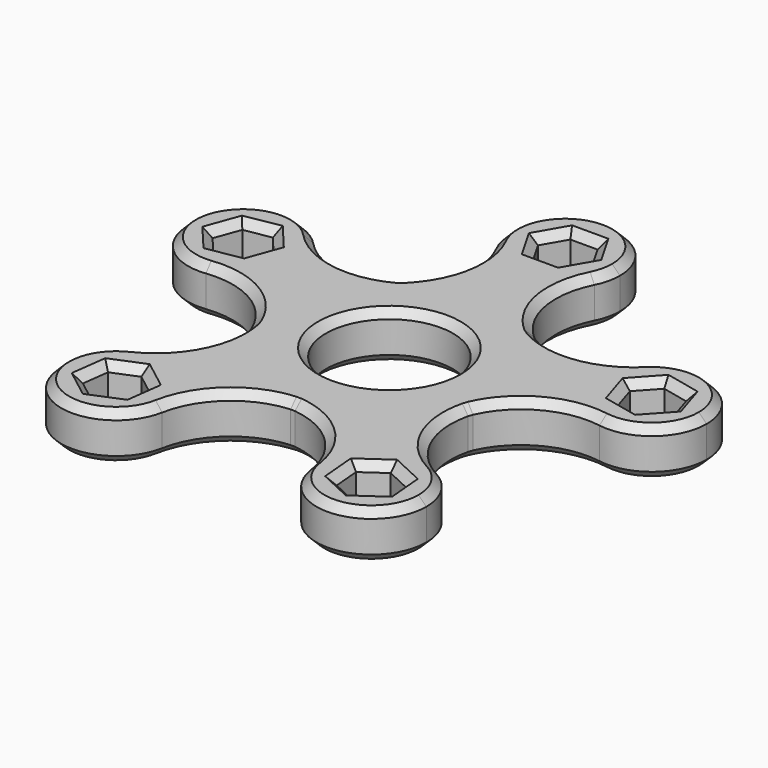
from build123d import *

# Parameters (mm, degrees)
F0_R        = 8.1
F1_DEPTH    = 6
F3_DEPTH    = 25
F4_C1_SIZE  = 1
F4_C2_SIZE  = 1
F4_C3_SIZE  = 1
F4_C4_SIZE  = 1
F4_C5_SIZE  = 1
F4_C6_SIZE  = 1
F4_C7_SIZE  = 1
F4_C8_SIZE  = 1
F4_C9_SIZE  = 1
F4_C10_SIZE = 1
F4_C11_SIZE = 1
F4_C12_SIZE = 1
F4_C13_SIZE = 1
F4_C14_SIZE = 1
F4_C15_SIZE = 1
F4_C16_SIZE = 1
F4_C17_SIZE = 1
F4_C18_SIZE = 1
F4_C19_SIZE = 1
F4_C20_SIZE = 1
F4_C21_SIZE = 1
F4_C22_SIZE = 1
F4_C23_SIZE = 1
F4_C24_SIZE = 1
F4_C25_SIZE = 1
F4_C26_SIZE = 1
F4_C27_SIZE = 1
F4_C28_SIZE = 1
F4_C29_SIZE = 1
F4_C30_SIZE = 1
F4_C31_SIZE = 1
F4_C32_SIZE = 1
F4_C33_SIZE = 1
F4_C34_SIZE = 1
F4_C35_SIZE = 1
F4_C36_SIZE = 1
F4_C37_SIZE = 1
F4_C38_SIZE = 1
F4_C39_SIZE = 1
F4_C40_SIZE = 1
F4_C41_SIZE = 1
F4_C42_SIZE = 1
F4_C43_SIZE = 1
F4_C44_SIZE = 1
F4_C45_SIZE = 1
F4_C46_SIZE = 1
F4_C47_SIZE = 1
F4_C48_SIZE = 1
F4_C49_SIZE = 1
F4_C50_SIZE = 1
F4_C51_SIZE = 1
F4_C52_SIZE = 1
F4_C53_SIZE = 1
F4_C54_SIZE = 1
F4_C55_SIZE = 1
F4_C56_SIZE = 1
F4_C57_SIZE = 1
F4_C58_SIZE = 1
F4_C59_SIZE = 1
F4_C60_SIZE = 1
F4_C61_SIZE = 1
F4_C62_SIZE = 0.9999
F4_C63_SIZE = 1
F4_C64_SIZE = 1
F4_C65_SIZE = 0.9999
F4_C66_SIZE = 0.9999
F4_C67_SIZE = 0.9999
F4_C68_SIZE = 0.9999
F4_C69_SIZE = 1
F4_C70_SIZE = 1
F4_C71_SIZE = 1
F4_C72_SIZE = 1
F4_C73_SIZE = 1
F4_C74_SIZE = 1
F4_C75_SIZE = 0.9999
F4_C76_SIZE = 0.9999
F4_C77_SIZE = 0.9999
F4_C78_SIZE = 0.9999
F4_C79_SIZE = 0.9999
F4_C80_SIZE = 0.9999


# Not quite as in the source:
# - a fillet or chamfer is up to 0.001 mm smaller than in the source, because OpenCascade refuses the exact size


with BuildPart() as f1:
    # F0 (on Top) → F1 (new body)
    with BuildSketch(Plane.XY):
        with BuildLine():
            ThreePointArc((14.2942212748, -4.5470032051), (14.8225051716, -2.3007260678), (15, 0))
            ThreePointArc((15, 0), (13.444632763, 6.6514547182), (9.1010866843, 11.9235154701))
            ThreePointArc((9.1010866843, 11.9235154701), (8.8696447255, 12.096669064), (8.6349092686, 12.2653308934))
            ThreePointArc((8.6349092686, 12.2653308934), (0.0381987951, 14.9999513617), (-8.5723280263, 12.3091507509))
            ThreePointArc((-8.5723280263, 12.3091507509), (-8.6036465453, 12.2872806643), (-8.6349092686, 12.2653308934))
            ThreePointArc((-8.6349092686, 12.2653308934), (-14.1084083641, 5.0943903887), (-14.4789538376, -3.9191702908))
            ThreePointArc((-14.4789538376, -3.9191702908), (-14.4007478158, -4.1974352105), (-14.3171944732, -4.4741415283))
            ThreePointArc((-14.3171944732, -4.4741415283), (-9.1314214351, -11.9003001044), (-0.6161262506, -14.9873409397))
            ThreePointArc((-0.6161262506, -14.9873409397), (-0.3272232755, -14.9964304062), (-0.0381987951, -14.9999513617))
            ThreePointArc((-0.0381987951, -14.9999513617), (8.6036465453, -12.2872806643), (14.1084083641, -5.0943903887))
            ThreePointArc((14.1084083641, -5.0943903887), (14.2039519424, -4.8215919795), (14.2942212748, -4.5470032051))
        make_face()
        Circle(F0_R, mode=Mode.SUBTRACT)
        with BuildLine():
            ThreePointArc((9.1010866843, 11.9235154701), (13.444632763, 6.6514547182), (15, 0))
            ThreePointArc((15, 0), (14.8225051716, -2.3007260678), (14.2942212748, -4.5470032051))
            ThreePointArc((14.2942212748, -4.5470032051), (18.9028221791, 0.3997534781), (25.5715973454, 1.5119772693))
            ThreePointArc((25.5715973454, 1.5119772693), (20.0280559657, 6.3148217896), (21.8142607752, 13.4287264061))
            ThreePointArc((21.8142607752, 13.4287264061), (15.7135746063, 10.5147545037), (9.1010866843, 11.9235154701))
        make_face()
        with BuildLine():
            ThreePointArc((-8.5723280263, 12.3091507509), (0.0381987951, 14.9999513617), (8.6349092686, 12.2653308934))
            ThreePointArc((8.6349092686, 12.2653308934), (5.302936588, 18.1481501185), (6.2475292735, 24.8427261796))
            ThreePointArc((6.2475292735, 24.8427261796), (0, 21), (-6.2475292735, 24.8427261796))
            ThreePointArc((-6.2475292735, 24.8427261796), (-5.2993669116, 18.1670506516), (-8.6062308953, 12.2909714987))
            ThreePointArc((-8.6062308953, 12.2909714987), (-8.589271136, 12.3000455997), (-8.5723280263, 12.3091507509))
        make_face()
        with BuildLine():
            ThreePointArc((33.704074621, 8.4197623861), (29.4217301436, 14.870680806), (21.8142607752, 13.4287264061))
            ThreePointArc((21.8142607752, 13.4287264061), (20.0280559657, 6.3148217896), (25.5715973454, 1.5119772693))
            ThreePointArc((25.5715973454, 1.5119772693), (31.2357773402, 3.0846269179), (33.704074621, 8.4197623861))
        make_face()
        with BuildLine():
            ThreePointArc((19.3668787275, -16.766534359), (14.7532626182, -11.8244547992), (14.1084083641, -5.0943903887))
            ThreePointArc((14.1084083641, -5.0943903887), (8.6036465453, -12.2872806643), (-0.0381987951, -14.9999513617))
            ThreePointArc((-0.0381987951, -14.9999513617), (6.0654399245, -17.90773374), (9.1315259752, -23.9334055124))
            ThreePointArc((9.1315259752, -23.9334055124), (12.0451051634, -17.2021929301), (19.3668787275, -16.766534359))
        make_face()
        with BuildLine():
            ThreePointArc((-8.6349092686, 12.2653308934), (-8.6036465453, 12.2872806643), (-8.5723280263, 12.3091507509))
            ThreePointArc((-8.5723280263, 12.3091507509), (-8.589271136, 12.3000455997), (-8.6062308953, 12.2909714987))
            ThreePointArc((-8.6062308953, 12.2909714987), (-8.6205583403, 12.2781380633), (-8.6349092686, 12.2653308934))
        make_face()
        with BuildLine():
            ThreePointArc((-6.2475292735, 24.8427261796), (0, 21), (6.2475292735, 24.8427261796))
            ThreePointArc((6.2475292735, 24.8427261796), (6.8092842838, 26.37714833), (7, 28))
            ThreePointArc((7, 28), (-1.62285167, 34.8092842838), (-6.2475292735, 24.8427261796))
        make_face()
        with BuildLine():
            ThreePointArc((23.0601402178, -22.9362572401), (22.0662691528, -19.3409248193), (19.3668787275, -16.766534359))
            ThreePointArc((19.3668787275, -16.766534359), (12.0451051634, -17.2021929301), (9.1315259752, -23.9334055124))
            ThreePointArc((9.1315259752, -23.9334055124), (16.5599903462, -29.9183879929), (23.0601402178, -22.9362572401))
        make_face()
        with BuildLine():
            ThreePointArc((-14.4789538376, -3.9191702908), (-14.1084083641, 5.0943903887), (-8.6349092686, 12.2653308934))
            ThreePointArc((-8.6349092686, 12.2653308934), (-8.6205583403, 12.2781380633), (-8.6062308953, 12.2909714987))
            ThreePointArc((-8.6062308953, 12.2909714987), (-15.2589532082, 11.1932732493), (-21.2077456136, 14.367469925))
            ThreePointArc((-21.2077456136, 14.367469925), (-19.8027247632, 12.1528467636), (-19.311393382, 9.5765640131))
            ThreePointArc((-19.311393382, 9.5765640131), (-21.0763861054, 4.9295543495), (-25.4813073287, 2.6259556121))
            ThreePointArc((-25.4813073287, 2.6259556121), (-18.8673938791, 1.2239025243), (-14.4789538376, -3.9191702908))
        make_face()
        with BuildLine():
            ThreePointArc((-10.1667952719, -23.5123146448), (-6.8407913445, -17.6261187719), (-0.6161262506, -14.9873409397))
            ThreePointArc((-0.6161262506, -14.9873409397), (-9.1314214351, -11.9003001044), (-14.3171944732, -4.4741415283))
            ThreePointArc((-14.3171944732, -4.4741415283), (-15.2549962555, -11.1696722613), (-20.0797917072, -15.9058049482))
            ThreePointArc((-20.0797917072, -15.9058049482), (-13.3198201709, -16.2876256526), (-10.0453200122, -22.2138935282))
            ThreePointArc((-10.0453200122, -22.2138935282), (-10.0757549906, -22.8659390854), (-10.1667952719, -23.5123146448))
        make_face()
        with BuildLine():
            ThreePointArc((-19.311393382, 9.5765640131), (-19.8027247632, 12.1528467636), (-21.2077456136, 14.367469925))
            ThreePointArc((-21.2077456136, 14.367469925), (-32.8892417275, 11.9707050164), (-25.4813073287, 2.6259556121))
            ThreePointArc((-25.4813073287, 2.6259556121), (-21.0763861054, 4.9295543495), (-19.311393382, 9.5765640131))
        make_face()
        with BuildLine():
            ThreePointArc((-20.0797917072, -15.9058049482), (-21.3066500153, -27.7673669102), (-10.1667952719, -23.5123146448))
            ThreePointArc((-10.1667952719, -23.5123146448), (-10.0757549906, -22.8659390854), (-10.0453200122, -22.2138935282))
            ThreePointArc((-10.0453200122, -22.2138935282), (-13.3198201709, -16.2876256526), (-20.0797917072, -15.9058049482))
        make_face()
    extrude(amount=F1_DEPTH)

    # F2 (on face) → F3 (cut)
    with BuildSketch(Plane.XY.offset(6)):
        Polygon((1.7320508076, 31), (-1.7320508076, 31), (-3.4641016151, 28), (-1.7320508076, 25), (1.7320508076, 25), (3.4641016151, 28), align=None)
        Polygon((30.0860631961, 7.6699935699), (29.0443877503, 10.9737659994), (25.6623991752, 11.7235348156), (23.3220860458, 9.1695312023), (24.3637614916, 5.8657587729), (27.7457500667, 5.1159899566), align=None)
        Polygon((16.362056567, -26.3871769027), (19.1996824867, -24.4002498432), (18.8977661375, -20.9493301805), (15.7582238686, -19.4853375774), (12.9205979489, -21.472264637), (13.2225142982, -24.9231842997), align=None)
        Polygon((-13.8449074315, -20.888239232), (-16.593164019, -18.7794277825), (-19.7935765997, -20.1050820787), (-20.245732593, -23.5395478243), (-17.4974760055, -25.6483592738), (-14.2970634248, -24.3227049776), align=None)
        Polygon((-24.0847117851, 6.9229082204), (-22.8999192542, 10.1780989458), (-25.1266008511, 12.8317547385), (-28.5380749789, 12.2302198058), (-29.7228675098, 8.9750290804), (-27.4961859129, 6.3213732877), align=None)
    extrude(amount=-F3_DEPTH, mode=Mode.SUBTRACT)

    # F4: chamfer of 1 on 100 edges, made by hand

    # F4_c1
    f4_c1_edges = [f1.edges().sort_by_distance(p)[0] for p in [
        (18.9028221791, 0.3997534781, 0),
        (33.3800932762, 10.5247029826, 0),
        (15.7135746063, 10.5147545037, 0),
    ]]
    chamfer(f4_c1_edges, length=F4_C1_SIZE)

    # F4_c2
    f4_c2_edges = [f1.edges().sort_by_distance(p)[0] for p in [
        (18.9028221791, 0.3997534781, 6),
        (33.3800932762, 10.5247029826, 6),
        (15.7135746063, 10.5147545037, 6),
    ]]
    chamfer(f4_c2_edges, length=F4_C2_SIZE)

    # F4_c3
    f4_c3_edges = [f1.edges().sort_by_distance(p)[0] for p in [
        (14.7532626182, -11.8244547992, 0),
        (20.0751752723, -28.6703215501, 0),
        (6.0654399245, -17.90773374, 0),
    ]]
    chamfer(f4_c3_edges, length=F4_C3_SIZE)

    # F4_c4
    f4_c4_edges = [f1.edges().sort_by_distance(p)[0] for p in [
        (5.302936588, 18.1481501185, 0),
        (0, 35, 0),
        (-5.2993669116, 18.1670506516, 0),
    ]]
    chamfer(f4_c4_edges, length=F4_C4_SIZE)

    # F4_c5
    f4_c5_edges = [f1.edges().sort_by_distance(p)[0] for p in [
        (-6.8407913445, -17.6261187719, 0),
        (-21.3066500153, -27.7673669102, 0),
        (-15.2549962555, -11.1696722613, 0),
    ]]
    chamfer(f4_c5_edges, length=F4_C5_SIZE)

    # F4_c6
    f4_c6_edges = [f1.edges().sort_by_distance(p)[0] for p in [
        (-15.2589532082, 11.1932732493, 0),
        (-32.8892417275, 11.9707050164, 0),
        (-18.8673938791, 1.2239025243, 0),
    ]]
    chamfer(f4_c6_edges, length=F4_C6_SIZE)

    # F4_c7
    f4_c7_edges = [f1.edges().sort_by_distance(p)[0] for p in [
        (-14.4007478158, -4.1974352105, 0),
    ]]
    chamfer(f4_c7_edges, length=F4_C7_SIZE)

    # F4_c8
    f4_c8_edges = [f1.edges().sort_by_distance(p)[0] for p in [
        (-15.8972697151, -24.9855321257, 0),
    ]]
    chamfer(f4_c8_edges, length=F4_C8_SIZE)

    # F4_c9
    f4_c9_edges = [f1.edges().sort_by_distance(p)[0] for p in [
        (-14.0709854281, -22.6054721048, 0),
    ]]
    chamfer(f4_c9_edges, length=F4_C9_SIZE)

    # F4_c10
    f4_c10_edges = [f1.edges().sort_by_distance(p)[0] for p in [
        (-15.2190357252, -19.8338335073, 0),
    ]]
    chamfer(f4_c10_edges, length=F4_C10_SIZE)

    # F4_c11
    f4_c11_edges = [f1.edges().sort_by_distance(p)[0] for p in [
        (-18.1933703093, -19.4422549306, 0),
    ]]
    chamfer(f4_c11_edges, length=F4_C11_SIZE)

    # F4_c12
    f4_c12_edges = [f1.edges().sort_by_distance(p)[0] for p in [
        (-20.0196545964, -21.8223149515, 0),
    ]]
    chamfer(f4_c12_edges, length=F4_C12_SIZE)

    # F4_c13
    f4_c13_edges = [f1.edges().sort_by_distance(p)[0] for p in [
        (-18.8716042993, -24.593953549, 0),
    ]]
    chamfer(f4_c13_edges, length=F4_C13_SIZE)

    # F4_c14
    f4_c14_edges = [f1.edges().sort_by_distance(p)[0] for p in [
        (-8.1, 0, 0),
    ]]
    chamfer(f4_c14_edges, length=F4_C14_SIZE)

    # F4_c15
    f4_c15_edges = [f1.edges().sort_by_distance(p)[0] for p in [
        (14.7922854326, -25.6551806012, 0),
    ]]
    chamfer(f4_c15_edges, length=F4_C15_SIZE)

    # F4_c16
    f4_c16_edges = [f1.edges().sort_by_distance(p)[0] for p in [
        (17.7808695269, -25.393713373, 0),
    ]]
    chamfer(f4_c16_edges, length=F4_C16_SIZE)

    # F4_c17
    f4_c17_edges = [f1.edges().sort_by_distance(p)[0] for p in [
        (19.0487243121, -22.6747900118, 0),
    ]]
    chamfer(f4_c17_edges, length=F4_C17_SIZE)

    # F4_c18
    f4_c18_edges = [f1.edges().sort_by_distance(p)[0] for p in [
        (17.3279950031, -20.217333879, 0),
    ]]
    chamfer(f4_c18_edges, length=F4_C18_SIZE)

    # F4_c19
    f4_c19_edges = [f1.edges().sort_by_distance(p)[0] for p in [
        (14.3394109088, -20.4788011072, 0),
    ]]
    chamfer(f4_c19_edges, length=F4_C19_SIZE)

    # F4_c20
    f4_c20_edges = [f1.edges().sort_by_distance(p)[0] for p in [
        (13.0715561236, -23.1977244683, 0),
    ]]
    chamfer(f4_c20_edges, length=F4_C20_SIZE)

    # F4_c21
    f4_c21_edges = [f1.edges().sort_by_distance(p)[0] for p in [
        (-28.6095267114, 7.6482011841, 0),
    ]]
    chamfer(f4_c21_edges, length=F4_C21_SIZE)

    # F4_c22
    f4_c22_edges = [f1.edges().sort_by_distance(p)[0] for p in [
        (-25.790448849, 6.6221407541, 0),
    ]]
    chamfer(f4_c22_edges, length=F4_C22_SIZE)

    # F4_c23
    f4_c23_edges = [f1.edges().sort_by_distance(p)[0] for p in [
        (-23.4923155196, 8.5505035831, 0),
    ]]
    chamfer(f4_c23_edges, length=F4_C23_SIZE)

    # F4_c24
    f4_c24_edges = [f1.edges().sort_by_distance(p)[0] for p in [
        (-24.0132600526, 11.5049268422, 0),
    ]]
    chamfer(f4_c24_edges, length=F4_C24_SIZE)

    # F4_c25
    f4_c25_edges = [f1.edges().sort_by_distance(p)[0] for p in [
        (-26.832337915, 12.5309872722, 0),
    ]]
    chamfer(f4_c25_edges, length=F4_C25_SIZE)

    # F4_c26
    f4_c26_edges = [f1.edges().sort_by_distance(p)[0] for p in [
        (-29.1304712444, 10.6026244431, 0),
    ]]
    chamfer(f4_c26_edges, length=F4_C26_SIZE)

    # F4_c27
    f4_c27_edges = [f1.edges().sort_by_distance(p)[0] for p in [
        (2.5980762114, 29.5, 0),
    ]]
    chamfer(f4_c27_edges, length=F4_C27_SIZE)

    # F4_c28
    f4_c28_edges = [f1.edges().sort_by_distance(p)[0] for p in [
        (0, 31, 0),
    ]]
    chamfer(f4_c28_edges, length=F4_C28_SIZE)

    # F4_c29
    f4_c29_edges = [f1.edges().sort_by_distance(p)[0] for p in [
        (-2.5980762114, 29.5, 0),
    ]]
    chamfer(f4_c29_edges, length=F4_C29_SIZE)

    # F4_c30
    f4_c30_edges = [f1.edges().sort_by_distance(p)[0] for p in [
        (-2.5980762114, 26.5, 0),
    ]]
    chamfer(f4_c30_edges, length=F4_C30_SIZE)

    # F4_c31
    f4_c31_edges = [f1.edges().sort_by_distance(p)[0] for p in [
        (0, 25, 0),
    ]]
    chamfer(f4_c31_edges, length=F4_C31_SIZE)

    # F4_c32
    f4_c32_edges = [f1.edges().sort_by_distance(p)[0] for p in [
        (2.5980762114, 26.5, 0),
    ]]
    chamfer(f4_c32_edges, length=F4_C32_SIZE)

    # F4_c33
    f4_c33_edges = [f1.edges().sort_by_distance(p)[0] for p in [
        (28.9159066314, 6.3929917633, 0),
    ]]
    chamfer(f4_c33_edges, length=F4_C33_SIZE)

    # F4_c34
    f4_c34_edges = [f1.edges().sort_by_distance(p)[0] for p in [
        (29.5652254732, 9.3218797846, 0),
    ]]
    chamfer(f4_c34_edges, length=F4_C34_SIZE)

    # F4_c35
    f4_c35_edges = [f1.edges().sort_by_distance(p)[0] for p in [
        (27.3533934628, 11.3486504075, 0),
    ]]
    chamfer(f4_c35_edges, length=F4_C35_SIZE)

    # F4_c36
    f4_c36_edges = [f1.edges().sort_by_distance(p)[0] for p in [
        (24.4922426105, 10.446533009, 0),
    ]]
    chamfer(f4_c36_edges, length=F4_C36_SIZE)

    # F4_c37
    f4_c37_edges = [f1.edges().sort_by_distance(p)[0] for p in [
        (23.8429237687, 7.5176449876, 0),
    ]]
    chamfer(f4_c37_edges, length=F4_C37_SIZE)

    # F4_c38
    f4_c38_edges = [f1.edges().sort_by_distance(p)[0] for p in [
        (26.0547557791, 5.4908743648, 0),
    ]]
    chamfer(f4_c38_edges, length=F4_C38_SIZE)

    # F4_c39
    f4_c39_edges = [f1.edges().sort_by_distance(p)[0] for p in [
        (14.7532626182, -11.8244547992, 6),
        (20.0751752723, -28.6703215501, 6),
        (6.0654399245, -17.90773374, 6),
    ]]
    chamfer(f4_c39_edges, length=F4_C39_SIZE)

    # F4_c40
    f4_c40_edges = [f1.edges().sort_by_distance(p)[0] for p in [
        (5.302936588, 18.1481501185, 6),
        (0, 35, 6),
        (-5.2993669116, 18.1670506516, 6),
    ]]
    chamfer(f4_c40_edges, length=F4_C40_SIZE)

    # F4_c41
    f4_c41_edges = [f1.edges().sort_by_distance(p)[0] for p in [
        (-6.8407913445, -17.6261187719, 6),
        (-21.3066500153, -27.7673669102, 6),
        (-15.2549962555, -11.1696722613, 6),
    ]]
    chamfer(f4_c41_edges, length=F4_C41_SIZE)

    # F4_c42
    f4_c42_edges = [f1.edges().sort_by_distance(p)[0] for p in [
        (-15.2589532082, 11.1932732493, 6),
        (-32.8892417275, 11.9707050164, 6),
        (-18.8673938791, 1.2239025243, 6),
    ]]
    chamfer(f4_c42_edges, length=F4_C42_SIZE)

    # F4_c43
    f4_c43_edges = [f1.edges().sort_by_distance(p)[0] for p in [
        (-14.4007478158, -4.1974352105, 6),
    ]]
    chamfer(f4_c43_edges, length=F4_C43_SIZE)

    # F4_c44
    f4_c44_edges = [f1.edges().sort_by_distance(p)[0] for p in [
        (-15.8972697151, -24.9855321257, 6),
    ]]
    chamfer(f4_c44_edges, length=F4_C44_SIZE)

    # F4_c45
    f4_c45_edges = [f1.edges().sort_by_distance(p)[0] for p in [
        (-14.0709854281, -22.6054721048, 6),
    ]]
    chamfer(f4_c45_edges, length=F4_C45_SIZE)

    # F4_c46
    f4_c46_edges = [f1.edges().sort_by_distance(p)[0] for p in [
        (-15.2190357252, -19.8338335073, 6),
    ]]
    chamfer(f4_c46_edges, length=F4_C46_SIZE)

    # F4_c47
    f4_c47_edges = [f1.edges().sort_by_distance(p)[0] for p in [
        (-18.1933703093, -19.4422549306, 6),
    ]]
    chamfer(f4_c47_edges, length=F4_C47_SIZE)

    # F4_c48
    f4_c48_edges = [f1.edges().sort_by_distance(p)[0] for p in [
        (-20.0196545964, -21.8223149515, 6),
    ]]
    chamfer(f4_c48_edges, length=F4_C48_SIZE)

    # F4_c49
    f4_c49_edges = [f1.edges().sort_by_distance(p)[0] for p in [
        (-18.8716042993, -24.593953549, 6),
    ]]
    chamfer(f4_c49_edges, length=F4_C49_SIZE)

    # F4_c50
    f4_c50_edges = [f1.edges().sort_by_distance(p)[0] for p in [
        (-8.1, 0, 6),
    ]]
    chamfer(f4_c50_edges, length=F4_C50_SIZE)

    # F4_c51
    f4_c51_edges = [f1.edges().sort_by_distance(p)[0] for p in [
        (14.7922854326, -25.6551806012, 6),
    ]]
    chamfer(f4_c51_edges, length=F4_C51_SIZE)

    # F4_c52
    f4_c52_edges = [f1.edges().sort_by_distance(p)[0] for p in [
        (17.7808695269, -25.393713373, 6),
    ]]
    chamfer(f4_c52_edges, length=F4_C52_SIZE)

    # F4_c53
    f4_c53_edges = [f1.edges().sort_by_distance(p)[0] for p in [
        (19.0487243121, -22.6747900118, 6),
    ]]
    chamfer(f4_c53_edges, length=F4_C53_SIZE)

    # F4_c54
    f4_c54_edges = [f1.edges().sort_by_distance(p)[0] for p in [
        (17.3279950031, -20.217333879, 6),
    ]]
    chamfer(f4_c54_edges, length=F4_C54_SIZE)

    # F4_c55
    f4_c55_edges = [f1.edges().sort_by_distance(p)[0] for p in [
        (14.3394109088, -20.4788011072, 6),
    ]]
    chamfer(f4_c55_edges, length=F4_C55_SIZE)

    # F4_c56
    f4_c56_edges = [f1.edges().sort_by_distance(p)[0] for p in [
        (13.0715561236, -23.1977244683, 6),
    ]]
    chamfer(f4_c56_edges, length=F4_C56_SIZE)

    # F4_c57
    f4_c57_edges = [f1.edges().sort_by_distance(p)[0] for p in [
        (-28.6095267114, 7.6482011841, 6),
    ]]
    chamfer(f4_c57_edges, length=F4_C57_SIZE)

    # F4_c58
    f4_c58_edges = [f1.edges().sort_by_distance(p)[0] for p in [
        (-25.790448849, 6.6221407541, 6),
    ]]
    chamfer(f4_c58_edges, length=F4_C58_SIZE)

    # F4_c59
    f4_c59_edges = [f1.edges().sort_by_distance(p)[0] for p in [
        (-23.4923155196, 8.5505035831, 6),
    ]]
    chamfer(f4_c59_edges, length=F4_C59_SIZE)

    # F4_c60
    f4_c60_edges = [f1.edges().sort_by_distance(p)[0] for p in [
        (-24.0132600526, 11.5049268422, 6),
    ]]
    chamfer(f4_c60_edges, length=F4_C60_SIZE)

    # F4_c61
    f4_c61_edges = [f1.edges().sort_by_distance(p)[0] for p in [
        (-26.832337915, 12.5309872722, 6),
    ]]
    chamfer(f4_c61_edges, length=F4_C61_SIZE)

    # F4_c62 (size 1 in the source; OpenCascade refuses exactly that, so slightly less here)
    f4_c62_edges = [f1.edges().sort_by_distance(p)[0] for p in [
        (-29.1304712444, 10.6026244431, 6),
    ]]
    chamfer(f4_c62_edges, length=F4_C62_SIZE)

    # F4_c63
    f4_c63_edges = [f1.edges().sort_by_distance(p)[0] for p in [
        (2.5980762114, 29.5, 6),
    ]]
    chamfer(f4_c63_edges, length=F4_C63_SIZE)

    # F4_c64
    f4_c64_edges = [f1.edges().sort_by_distance(p)[0] for p in [
        (0, 31, 6),
    ]]
    chamfer(f4_c64_edges, length=F4_C64_SIZE)

    # F4_c65 (size 1 in the source; OpenCascade refuses exactly that, so slightly less here)
    f4_c65_edges = [f1.edges().sort_by_distance(p)[0] for p in [
        (-2.5980762114, 29.5, 6),
    ]]
    chamfer(f4_c65_edges, length=F4_C65_SIZE)

    # F4_c66 (size 1 in the source; OpenCascade refuses exactly that, so slightly less here)
    f4_c66_edges = [f1.edges().sort_by_distance(p)[0] for p in [
        (-2.5980762114, 26.5, 6),
    ]]
    chamfer(f4_c66_edges, length=F4_C66_SIZE)

    # F4_c67 (size 1 in the source; OpenCascade refuses exactly that, so slightly less here)
    f4_c67_edges = [f1.edges().sort_by_distance(p)[0] for p in [
        (0, 25, 6),
    ]]
    chamfer(f4_c67_edges, length=F4_C67_SIZE)

    # F4_c68 (size 1 in the source; OpenCascade refuses exactly that, so slightly less here)
    f4_c68_edges = [f1.edges().sort_by_distance(p)[0] for p in [
        (2.5980762114, 26.5, 6),
    ]]
    chamfer(f4_c68_edges, length=F4_C68_SIZE)

    # F4_c69
    f4_c69_edges = [f1.edges().sort_by_distance(p)[0] for p in [
        (28.9159066314, 6.3929917633, 6),
    ]]
    chamfer(f4_c69_edges, length=F4_C69_SIZE)

    # F4_c70
    f4_c70_edges = [f1.edges().sort_by_distance(p)[0] for p in [
        (29.5652254732, 9.3218797846, 6),
    ]]
    chamfer(f4_c70_edges, length=F4_C70_SIZE)

    # F4_c71
    f4_c71_edges = [f1.edges().sort_by_distance(p)[0] for p in [
        (27.3533934628, 11.3486504075, 6),
    ]]
    chamfer(f4_c71_edges, length=F4_C71_SIZE)

    # F4_c72
    f4_c72_edges = [f1.edges().sort_by_distance(p)[0] for p in [
        (24.4922426105, 10.446533009, 6),
    ]]
    chamfer(f4_c72_edges, length=F4_C72_SIZE)

    # F4_c73
    f4_c73_edges = [f1.edges().sort_by_distance(p)[0] for p in [
        (23.8429237687, 7.5176449876, 6),
    ]]
    chamfer(f4_c73_edges, length=F4_C73_SIZE)

    # F4_c74
    f4_c74_edges = [f1.edges().sort_by_distance(p)[0] for p in [
        (26.0547557791, 5.4908743648, 6),
    ]]
    chamfer(f4_c74_edges, length=F4_C74_SIZE)

    # F4_c75 (size 1 in the source; OpenCascade refuses exactly that, so slightly less here)
    f4_c75_edges = [f1.edges().sort_by_distance(p)[0] for p in [
        (14.2039519424, -4.8215919795, 0),
    ]]
    chamfer(f4_c75_edges, length=F4_C75_SIZE)

    # F4_c76 (size 1 in the source; OpenCascade refuses exactly that, so slightly less here)
    f4_c76_edges = [f1.edges().sort_by_distance(p)[0] for p in [
        (14.2039519424, -4.8215919795, 6),
    ]]
    chamfer(f4_c76_edges, length=F4_C76_SIZE)

    # F4_c77 (size 1 in the source; OpenCascade refuses exactly that, so slightly less here)
    f4_c77_edges = [f1.edges().sort_by_distance(p)[0] for p in [
        (8.8696447255, 12.096669064, 0),
    ]]
    chamfer(f4_c77_edges, length=F4_C77_SIZE)

    # F4_c78 (size 1 in the source; OpenCascade refuses exactly that, so slightly less here)
    f4_c78_edges = [f1.edges().sort_by_distance(p)[0] for p in [
        (-0.3272232755, -14.9964304062, 0),
    ]]
    chamfer(f4_c78_edges, length=F4_C78_SIZE)

    # F4_c79 (size 1 in the source; OpenCascade refuses exactly that, so slightly less here)
    f4_c79_edges = [f1.edges().sort_by_distance(p)[0] for p in [
        (8.8696447255, 12.096669064, 6),
    ]]
    chamfer(f4_c79_edges, length=F4_C79_SIZE)

    # F4_c80 (size 1 in the source; OpenCascade refuses exactly that, so slightly less here)
    f4_c80_edges = [f1.edges().sort_by_distance(p)[0] for p in [
        (-0.3272232755, -14.9964304062, 6),
    ]]
    chamfer(f4_c80_edges, length=F4_C80_SIZE)


solid = f1.part
